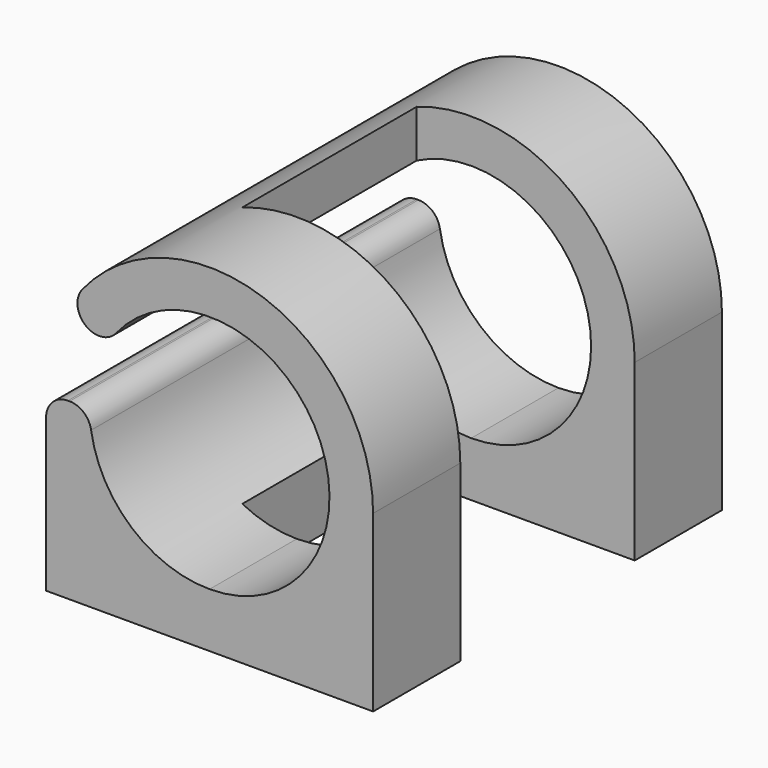
from build123d import *

# Parameters (mm, degrees)
F0_W         = 19.05
F0_H         = 25.4
F1_DEPTH     = 3.175
F3_DEPTH     = 25.4
F4_R         = 1.26999
F5_W         = 12.7
F5_H         = 12.7
F6_DEPTH     = 19.686
F7_TEXT_SIZE = 8.3332051775
F8_DEPTH     = 1.27


# Not quite as in the source:
# - a fillet or chamfer is up to 0.001 mm smaller than in the source, because OpenCascade refuses the exact size
# - Text() gives the source's letters only with a copy of the font that has no kerning and outlines rounded to 1/6400 em; it was checked with that copy


with BuildPart() as f1:
    # F0 (on Top) → F1 (new body)
    with BuildSketch(Plane.XY):
        with Locations((9.525, 12.7)):
            Rectangle(F0_W, F0_H)
    extrude(amount=F1_DEPTH)

    # F2 (on face) → F3 (join, through all)
    with BuildSketch(Plane.XZ):
        with BuildLine():
            Line((9.525, 3.175), (19.05, 3.175))
            Line((19.05, 3.175), (19.05, 10.16))
            ThreePointArc((19.05, 10.16), (11.9902514046, 19.3604434954), (1.276108029, 14.9225))
            Line((1.276108029, 14.9225), (3.4758125546, 13.6525))
            ThreePointArc((3.4758125546, 13.6525), (15.5741874454, 13.6525), (9.525, 3.175))
        make_face()
        with BuildLine():
            Line((0, 3.175), (9.525, 3.175))
            ThreePointArc((9.525, 3.175), (4.5858591334, 5.2208591334), (2.54, 10.16))
            Line((2.54, 10.16), (0, 10.16))
            Line((0, 10.16), (0, 3.175))
        make_face()
    extrude(amount=-F3_DEPTH)

    # F4 (radius 1.27 in the source; OpenCascade refuses exactly that, so slightly less here)
    f4_edges = [f1.edges().sort_by_distance(p)[0] for p in [
        (1.276108, 12.7, 14.9225),
        (3.475813, 12.7, 13.6525),
        (2.54, 12.7, 10.16),
        (0, 12.7, 10.16),
    ]]
    fillet(f4_edges, radius=F4_R)

    # F5 (on face) → F6 (cut, through all)
    with BuildSketch(Plane(origin=(0, 0, 0), x_dir=(1, 0, 0), z_dir=(0, 0, -1))):
        with Locations((12.7, -12.7)):
            Rectangle(F5_W, F5_H)
    extrude(amount=-F6_DEPTH, mode=Mode.SUBTRACT)

    # F7 (on face) → F8 (cut)
    with BuildSketch(Plane(origin=(0, 0, 0), x_dir=(0, -1, 0), z_dir=(-1, 0, 0))):
        with Locations((-17.78, 1.6200922722)):
            Text('TC', F7_TEXT_SIZE, font='Open Sans', text_align=(TextAlign.LEFT, TextAlign.BOTTOM))
    extrude(amount=-F8_DEPTH, mode=Mode.SUBTRACT)


solid = f1.part
